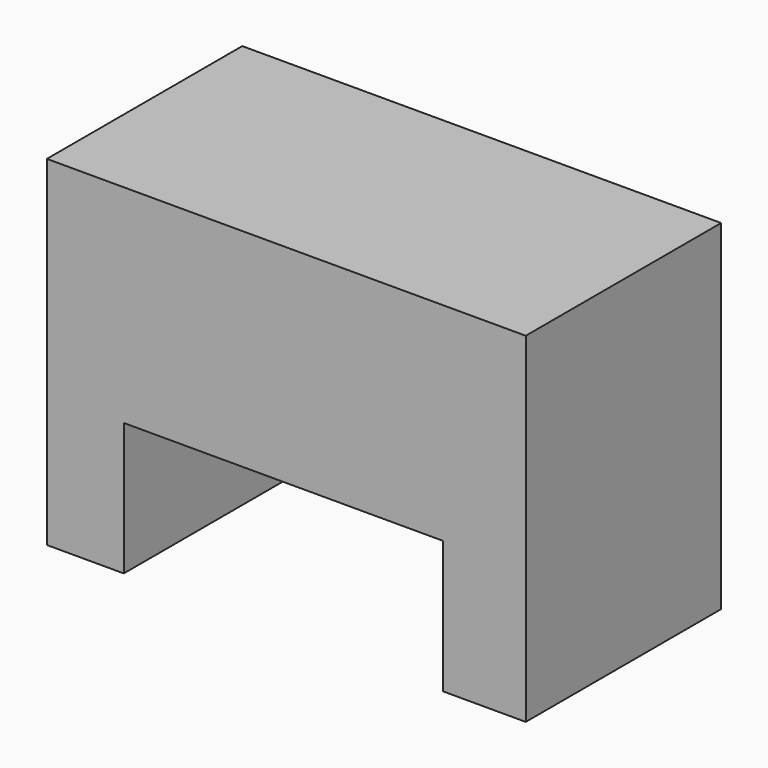
from build123d import *

# Parameters (mm, degrees)
F1_DEPTH = 50.8


# Not quite as in the source:
# - the program builds the solid bodies; features that only make, move or delete a surface that nothing else refers to are left out


with BuildPart() as f1:
    # F0 (on Front) → F1 (new body)
    with BuildSketch(Plane.XZ):
        Polygon((57.1499988437, 23.2726577669), (-42.4610599875, 23.2726577669), (-42.4610599875, -47.4423281848), (-26.4612324536, -47.4423281848), (-26.4612324536, -19.8850687593), (39.9267114699, -19.8850687593), (39.9267114699, -47.4423281848), (57.1499988437, -47.4423281848), align=None)
    extrude(amount=F1_DEPTH)


solid = f1.part
